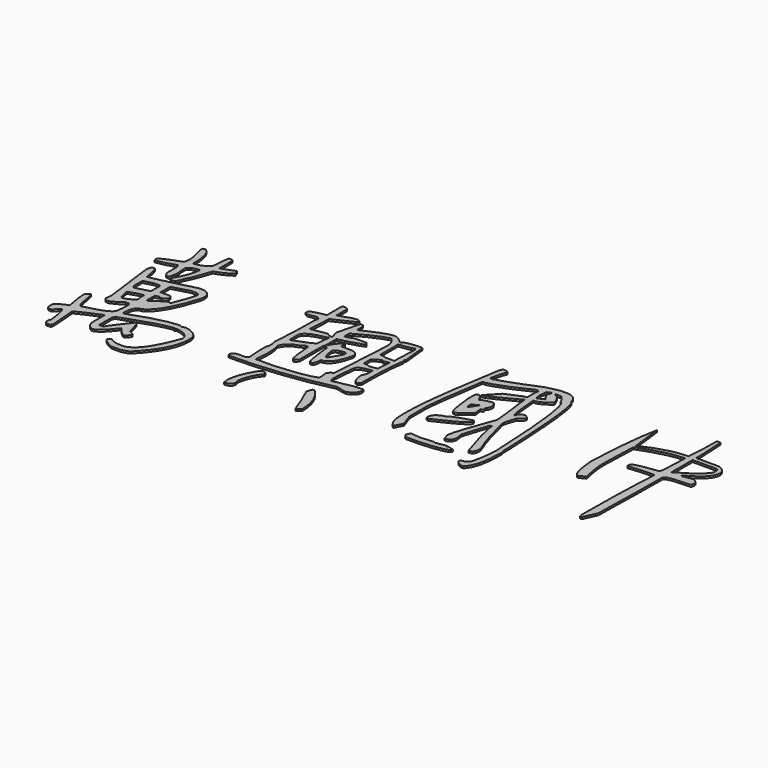
from build123d import *

# Parameters (mm, degrees)
F1_DEPTH = 1


# Not quite as in the source:
# - ends of sketch curves that miss each other by under 0.0002 mm in the source are joined


with BuildPart() as f1:
    # F0 (on Top) → F1 (new body)
    with BuildSketch(Plane.XY):
        with BuildLine():
            Line((-129.622072, 32.734284), (-130.536865, 32.734284))
            add(Edge.make_bspline(
                [(-134.633542, 45.790156), (-131.902424, 44.52872), (-130.536865, 40.176762), (-130.536865, 32.734284)],
                knots=[0, 0, 0, 0, 1, 1, 1, 1], degree=3))
            add(Edge.make_bspline(
                [(-135.786971, 45.269817), (-135.62788, 45.269817), (-135.243404, 45.443263), (-134.633542, 45.790156)],
                knots=[0, 0, 0, 0, 1, 1, 1, 1], degree=3))
            Line((-135.786971, 45.269817), (-135.786971, 44.560262))
            add(Edge.make_bspline(
                [(-133.758523, 34.910264), (-133.758523, 35.604054), (-134.434672, 38.82072), (-135.786971, 44.560262)],
                knots=[0, 0, 0, 0, 1, 1, 1, 1], degree=3))
            Line((-133.758523, 34.910264), (-134.315351, 31.598998))
            add(Edge.make_bspline(
                [(-144.815578, 26.584786), (-144.815578, 27.467788), (-141.315502, 29.139192), (-134.315351, 31.598998)],
                knots=[0, 0, 0, 0, 1, 1, 1, 1], degree=3))
            Line((-144.815578, 26.584786), (-144.815578, 25.307579))
            add(Edge.make_bspline(
                [(-134.474446, 27.767376), (-139.03515, 26.127512), (-142.482194, 25.307579), (-144.815578, 25.307579)],
                knots=[0, 0, 0, 0, 1, 1, 1, 1], degree=3))
            Line((-134.474446, 27.767376), (-133.758523, 26.111743))
            Line((-133.758523, 26.111743), (-133.758523, 19.583812))
            add(Edge.make_bspline(
                [(-132.167581, 17.50244), (-132.538799, 17.50244), (-133.069113, 18.196231), (-133.758523, 19.583812)],
                knots=[0, 0, 0, 0, 1, 1, 1, 1], degree=3))
            Line((-132.167581, 17.50244), (-131.133466, 17.50244))
            add(Edge.make_bspline(
                [(-130.059578, 22.374739), (-130.351253, 19.12654), (-130.709216, 17.50244), (-131.133466, 17.50244)],
                knots=[0, 0, 0, 0, 1, 1, 1, 1], degree=3))
            add(Edge.make_bspline(
                [(-130.536865, 27.199734), (-130.536865, 25.528333), (-130.377769, 23.920001), (-130.059578, 22.374739)],
                knots=[0, 0, 0, 0, 1, 1, 1, 1], degree=3))
            add(Edge.make_bspline(
                [(-124.650376, 30.179878), (-128.574702, 29.580696), (-130.536865, 28.587315), (-130.536865, 27.199734)],
                knots=[0, 0, 0, 0, 1, 1, 1, 1], degree=3))
            add(Edge.make_bspline(
                [(-129.264107, 17.50244), (-126.692084, 21.507502), (-125.154174, 25.733315), (-124.650376, 30.179878)],
                knots=[0, 0, 0, 0, 1, 1, 1, 1], degree=3))
            Line((-129.264107, 17.50244), (-129.264107, 16.367146))
            add(Edge.make_bspline(
                [(-128.03113, 15.752199), (-128.667503, 16.162163), (-129.078495, 16.367146), (-129.264107, 16.367146)],
                knots=[0, 0, 0, 0, 1, 1, 1, 1], degree=3))
            add(Edge.make_bspline(
                [(-124.96856, 19.631116), (-125.604938, 17.045171), (-126.625794, 15.752199), (-128.03113, 15.752199)],
                knots=[0, 0, 0, 0, 1, 1, 1, 1], degree=3))
            add(Edge.make_bspline(
                [(-119.877542, 32.355858), (-121.945771, 26.080207), (-123.642777, 21.838627), (-124.96856, 19.631116)],
                knots=[0, 0, 0, 0, 1, 1, 1, 1], degree=3))
            add(Edge.make_bspline(
                [(-111.485318, 36.471297), (-114.136893, 34.579143), (-116.934301, 33.20733), (-119.877542, 32.355858)],
                knots=[0, 0, 0, 0, 1, 1, 1, 1], degree=3))
            Line((-111.485318, 36.471297), (-112.280789, 38.694573))
            add(Edge.make_bspline(
                [(-119.519584, 36.092863), (-115.117976, 37.827336), (-112.705044, 38.694573), (-112.280789, 38.694573)],
                knots=[0, 0, 0, 0, 1, 1, 1, 1], degree=3))
            Line((-119.519584, 36.092863), (-119.519584, 44.512957))
            add(Edge.make_bspline(
                [(-120.155959, 45.269817), (-119.731709, 45.175209), (-119.519584, 44.922922), (-119.519584, 44.512957)],
                knots=[0, 0, 0, 0, 1, 1, 1, 1], degree=3))
            Line((-120.155959, 45.269817), (-121.62758, 45.269817))
            add(Edge.make_bspline(
                [(-122.701468, 37.37007), (-122.489341, 42.636568), (-122.131378, 45.269817), (-121.62758, 45.269817)],
                knots=[0, 0, 0, 0, 1, 1, 1, 1], degree=3))
            add(Edge.make_bspline(
                [(-129.622072, 32.734284), (-125.008336, 33.7119), (-122.701468, 35.257162), (-122.701468, 37.37007)],
                knots=[0, 0, 0, 0, 1, 1, 1, 1], degree=3))
        make_face()
    extrude(amount=F1_DEPTH)


with BuildPart() as f1b:
    # F0 (on Top) → F1, piece 2 (new body)
    with BuildSketch(Plane.XY):
        with BuildLine():
            Line((-140.20184, 19.583812), (-141.19618, 19.583812))
            add(Edge.make_bspline(
                [(-142.309843, 17.029397), (-141.93862, 18.73234), (-141.567399, 19.583812), (-141.19618, 19.583812)],
                knots=[0, 0, 0, 0, 1, 1, 1, 1], degree=3))
            Line((-142.309843, 17.029397), (-138.809767, -10.40685))
            Line((-138.809767, -10.40685), (-139.287047, -13.386994))
            add(Edge.make_bspline(
                [(-136.701764, -14.711506), (-138.213163, -14.711506), (-139.074924, -14.270002), (-139.287047, -13.386994)],
                knots=[0, 0, 0, 0, 1, 1, 1, 1], degree=3))
            Line((-136.701764, -14.711506), (-132.741804248, -12.6892637488))
            Line((-132.741804248, -12.6892637488), (-130.775501, -11.116414))
            Line((-130.775501, -11.116414), (-129.661846, -11.116414))
            add(Edge.make_bspline(
                [(-128.269766, -12.819351), (-128.269766, -11.68406), (-128.733793, -11.116414), (-129.661846, -11.116414)],
                knots=[0, 0, 0, 0, 1, 1, 1, 1], degree=3))
            Line((-128.269766, -12.819351), (-128.269766, -13.386994))
            add(Edge.make_bspline(
                [(-128.747053, -18.826945), (-128.428862, -16.682501), (-128.269766, -14.869184), (-128.269766, -13.386994)],
                knots=[0, 0, 0, 0, 1, 1, 1, 1], degree=3))
            add(Edge.make_bspline(
                [(-142.826896, -25.260268), (-133.440334, -23.241969), (-128.747053, -21.097527), (-128.747053, -18.826945)],
                knots=[0, 0, 0, 0, 1, 1, 1, 1], degree=3))
            Line((-142.826896, -25.260268), (-144.059873, -23.793852))
            add(Edge.make_bspline(
                [(-146.20765, -14.474984), (-145.756884, -14.474984), (-145.040959, -17.581274), (-144.059873, -23.793852)],
                knots=[0, 0, 0, 0, 1, 1, 1, 1], degree=3))
            Line((-146.20765, -14.474984), (-148.315646, -15.799496))
            add(Edge.make_bspline(
                [(-146.764478, -27.436248), (-147.79859, -22.422039), (-148.315646, -18.543122), (-148.315646, -15.799496)],
                knots=[0, 0, 0, 0, 1, 1, 1, 1], degree=3))
            add(Edge.make_bspline(
                [(-152.849837, -31.362469), (-152.637709, -30.227178), (-150.609256, -28.918437), (-146.764478, -27.436248)],
                knots=[0, 0, 0, 0, 1, 1, 1, 1], degree=3))
            Line((-152.849837, -31.362469), (-152.849837, -33.680362))
            add(Edge.make_bspline(
                [(-150.383875, -35.004874), (-151.815722, -35.004874), (-152.637709, -34.56337), (-152.849837, -33.680362)],
                knots=[0, 0, 0, 0, 1, 1, 1, 1], degree=3))
            Line((-150.383875, -35.004874), (-147.400861, -32.02473))
            add(Edge.make_bspline(
                [(-144.775804, -42.526187), (-145.491725, -35.525215), (-146.366744, -32.02473), (-147.400861, -32.02473)],
                knots=[0, 0, 0, 0, 1, 1, 1, 1], degree=3))
            add(Edge.make_bspline(
                [(-145.332631, -42.6681), (-145.332631, -42.573491), (-145.147022, -42.526187), (-144.775804, -42.526187)],
                knots=[0, 0, 0, 0, 1, 1, 1, 1], degree=3))
            Line((-145.332631, -42.6681), (-145.332631, -44.371037))
            add(Edge.make_bspline(
                [(-144.218969, -45.790157), (-144.53716, -45.790157), (-144.908381, -45.317117), (-145.332631, -44.371037)],
                knots=[0, 0, 0, 0, 1, 1, 1, 1], degree=3))
            Line((-144.218969, -45.790157), (-142.071199, -45.790157))
            add(Edge.make_bspline(
                [(-141.593912, -44.371037), (-141.912104, -45.1279), (-142.071199, -45.60094), (-142.071199, -45.790157)],
                knots=[0, 0, 0, 0, 1, 1, 1, 1], degree=3))
            add(Edge.make_bspline(
                [(-142.628027, -30.842131), (-141.938617, -38.221537), (-141.593912, -42.731172), (-141.593912, -44.371037)],
                knots=[0, 0, 0, 0, 1, 1, 1, 1], degree=3))
            Line((-142.628027, -30.842131), (-142.071199, -30.842131))
            add(Edge.make_bspline(
                [(-130.258447, -25.260268), (-138.133615, -28.571539), (-142.071199, -30.43216), (-142.071199, -30.842131)],
                knots=[0, 0, 0, 0, 1, 1, 1, 1], degree=3))
            Line((-130.258447, -25.260268), (-130.258447, -32.497764))
            add(Edge.make_bspline(
                [(-127.036789, -37.985018), (-129.184561, -36.912794), (-130.258447, -35.083709), (-130.258447, -32.497764)],
                knots=[0, 0, 0, 0, 1, 1, 1, 1], degree=3))
            add(Edge.make_bspline(
                [(-117.61045, -29.990662), (-121.587808, -35.320233), (-124.729921, -37.985018), (-127.036789, -37.985018)],
                knots=[0, 0, 0, 0, 1, 1, 1, 1], degree=3))
            add(Edge.make_bspline(
                [(-112.638754, -34.389918), (-113.858478, -34.389918), (-115.51571, -32.9235), (-117.61045, -29.990662)],
                knots=[0, 0, 0, 0, 1, 1, 1, 1], degree=3))
            Line((-112.638754, -34.389918), (-110.451211, -31.882817))
            add(Edge.make_bspline(
                [(-113.394452, -29.848749), (-111.432291, -30.889432), (-110.451211, -31.567455), (-110.451211, -31.882817)],
                knots=[0, 0, 0, 0, 1, 1, 1, 1], degree=3))
            add(Edge.make_bspline(
                [(-115.621769, -22.80047), (-115.224035, -22.80047), (-114.481596, -25.149897), (-113.394452, -29.848749)],
                knots=[0, 0, 0, 0, 1, 1, 1, 1], degree=3))
            Line((-115.621769, -22.80047), (-116.41724, -22.80047))
            add(Edge.make_bspline(
                [(-124.212863, -33.585754), (-124.212863, -32.828891), (-121.614322, -29.233796), (-116.41724, -22.80047)],
                knots=[0, 0, 0, 0, 1, 1, 1, 1], degree=3))
            Line((-124.212863, -33.585754), (-126.559502, -33.585754))
            Line((-126.559502, -33.585754), (-126.559502, -25.260268))
            Line((-126.559502, -25.260268), (-125.923127, -23.793852))
            add(Edge.make_bspline(
                [(-100.627133, -16.509052), (-104.074177, -16.509052), (-112.506175, -18.937318), (-125.923127, -23.793852)],
                knots=[0, 0, 0, 0, 1, 1, 1, 1], degree=3))
            Line((-100.627133, -16.509052), (-100.627133, -17.076703))
            add(Edge.make_bspline(
                [(-99.593026, -16.509052), (-100.255914, -16.887486), (-100.600617, -17.076703), (-100.627133, -17.076703)],
                knots=[0, 0, 0, 0, 1, 1, 1, 1], degree=3))
            add(Edge.make_bspline(
                [(-92.592874, -21.807089), (-92.592874, -18.968855), (-94.926258, -17.202842), (-99.593026, -16.509052)],
                knots=[0, 0, 0, 0, 1, 1, 1, 1], degree=3))
            add(Edge.make_bspline(
                [(-108.06479, -41.958544), (-102.523006, -41.958544), (-97.365701, -35.241393), (-92.592874, -21.807089)],
                knots=[0, 0, 0, 0, 1, 1, 1, 1], degree=3))
            add(Edge.make_bspline(
                [(-114.66721, -40.113686), (-113.049747, -41.343591), (-110.84894, -41.958544), (-108.06479, -41.958544)],
                knots=[0, 0, 0, 0, 1, 1, 1, 1], degree=3))
            add(Edge.make_bspline(
                [(-116.178604, -41.438197), (-116.178604, -40.744407), (-115.674806, -40.302903), (-114.66721, -40.113686)],
                knots=[0, 0, 0, 0, 1, 1, 1, 1], degree=3))
            add(Edge.make_bspline(
                [(-111.008038, -45.175202), (-114.216439, -43.693018), (-115.93996, -42.44735), (-116.178604, -41.438197)],
                knots=[0, 0, 0, 0, 1, 1, 1, 1], degree=3))
            Line((-111.008038, -45.175202), (-106.553396, -45.175202))
            add(Edge.make_bspline(
                [(-102.218075, -44.039907), (-104.286304, -44.79677), (-105.731411, -45.175202), (-106.553396, -45.175202)],
                knots=[0, 0, 0, 0, 1, 1, 1, 1], degree=3))
            add(Edge.make_bspline(
                [(-89.888269, -20.577186), (-89.888269, -27.956592), (-93.998205, -35.777499), (-102.218075, -44.039907)],
                knots=[0, 0, 0, 0, 1, 1, 1, 1], degree=3))
            Line((-89.888269, -20.577186), (-89.888269, -19.962239))
            add(Edge.make_bspline(
                [(-97.56457, -13.292386), (-92.447036, -14.270002), (-89.888269, -16.493286), (-89.888269, -19.962239)],
                knots=[0, 0, 0, 0, 1, 1, 1, 1], degree=3))
            add(Edge.make_bspline(
                [(-98.996417, -13.907341), (-98.307012, -13.497371), (-97.82973, -13.292386), (-97.56457, -13.292386)],
                knots=[0, 0, 0, 0, 1, 1, 1, 1], degree=3))
            add(Edge.make_bspline(
                [(-100.547585, -13.292386), (-100.229399, -13.292386), (-99.712342, -13.497371), (-98.996417, -13.907341)],
                knots=[0, 0, 0, 0, 1, 1, 1, 1], degree=3))
            add(Edge.make_bspline(
                [(-124.531054, -19.252674), (-113.686124, -15.279149), (-105.691635, -13.292386), (-100.547585, -13.292386)],
                knots=[0, 0, 0, 0, 1, 1, 1, 1], degree=3))
            Line((-124.531054, -19.252674), (-125.525395, -19.252674))
            add(Edge.make_bspline(
                [(-121.707128, -11.731361), (-124.252639, -11.731361), (-125.525395, -14.238466), (-125.525395, -19.252674)],
                knots=[0, 0, 0, 0, 1, 1, 1, 1], degree=3))
            add(Edge.make_bspline(
                [(-108.462529, 11.211021), (-112.174728, -1.403347), (-116.589594, -9.050808), (-121.707128, -11.731361)],
                knots=[0, 0, 0, 0, 1, 1, 1, 1], degree=3))
            Line((-108.462529, 11.211021), (-108.462529, 12.299011))
            add(Edge.make_bspline(
                [(-112.59898, 17.17131), (-109.841346, 16.698273), (-108.462529, 15.074173), (-108.462529, 12.299011)],
                knots=[0, 0, 0, 0, 1, 1, 1, 1], degree=3))
            Line((-112.59898, 17.17131), (-115.064942, 17.17131))
            add(Edge.make_bspline(
                [(-138.014296, 11.825968), (-136.396838, 11.825968), (-128.747053, 13.607749), (-115.064942, 17.17131)],
                knots=[0, 0, 0, 0, 1, 1, 1, 1], degree=3))
            add(Edge.make_bspline(
                [(-140.20184, 19.583812), (-139.432882, 19.583812), (-138.703701, 16.997864), (-138.014296, 11.825968)],
                knots=[0, 0, 0, 0, 1, 1, 1, 1], degree=3))
        make_face()
        with BuildLine():
            add(Edge.make_bspline(
                [(-136.105162, -3.547788), (-135.574848, -7.237494), (-134.911955, -9.082347), (-134.116481, -9.082347)],
                knots=[0, 0, 0, 0, 1, 1, 1, 1], degree=3))
            add(Edge.make_bspline(
                [(-128.747053, -1.561025), (-129.860713, -1.561025), (-132.313416, -2.223279), (-136.105162, -3.547788)],
                knots=[0, 0, 0, 0, 1, 1, 1, 1], degree=3))
            add(Edge.make_bspline(
                [(-128.150444, -5.676464), (-128.548183, -4.951137), (-128.747053, -3.579324), (-128.747053, -1.561025)],
                knots=[0, 0, 0, 0, 1, 1, 1, 1], degree=3))
            add(Edge.make_bspline(
                [(-134.116481, -9.082347), (-131.305815, -8.293948), (-129.317136, -7.158653), (-128.150444, -5.676464)],
                knots=[0, 0, 0, 0, 1, 1, 1, 1], degree=3))
        make_face(mode=Mode.SUBTRACT)
        with BuildLine():
            Line((-137.099503, 2.696327), (-137.099503, 7.899747))
            Line((-137.099503, 7.899747), (-132.207355, 9.176954))
            Line((-132.207355, 9.176954), (-128.747053, 9.176954))
            Line((-128.747053, 9.176954), (-128.747053, 2.980144))
            Line((-128.747053, 2.980144), (-135.627883, 1.040685))
            add(Edge.make_bspline(
                [(-137.099503, 2.696327), (-136.913892, 1.592566), (-136.423351, 1.040685), (-135.627883, 1.040685)],
                knots=[0, 0, 0, 0, 1, 1, 1, 1], degree=3))
        make_face(mode=Mode.SUBTRACT)
        with BuildLine():
            Line((-125.008334, 4.635785), (-125.008334, 10.879891))
            Line((-125.008334, 10.879891), (-116.099056, 13.339697))
            Line((-116.099056, 13.339697), (-112.99672, 13.339697))
            Line((-112.99672, 13.339697), (-111.684188, 12.582837))
            add(Edge.make_bspline(
                [(-115.820639, -0.141914), (-113.063005, 6.669847), (-111.684188, 10.91143), (-111.684188, 12.582837)],
                knots=[0, 0, 0, 0, 1, 1, 1, 1], degree=3))
            Line((-115.820639, -0.141914), (-117.61045, -0.141914))
            add(Edge.make_bspline(
                [(-124.013993, -4.351952), (-120.222247, -1.54526), (-118.087733, -0.141914), (-117.61045, -0.141914)],
                knots=[0, 0, 0, 0, 1, 1, 1, 1], degree=3))
            Line((-124.013993, -4.351952), (-125.008334, -4.351952))
            Line((-125.008334, -4.351952), (-125.008334, 0.804172))
            add(Edge.make_bspline(
                [(-123.099208, 1.466424), (-123.815128, 1.024923), (-124.451504, 0.804172), (-125.008334, 0.804172)],
                knots=[0, 0, 0, 0, 1, 1, 1, 1], degree=3))
            Line((-123.099208, 1.466424), (-122.025319, 0.804172))
            add(Edge.make_bspline(
                [(-119.002523, 2.838231), (-119.453294, 1.482192), (-120.460893, 0.804172), (-122.025319, 0.804172)],
                knots=[0, 0, 0, 0, 1, 1, 1, 1], degree=3))
            Line((-119.002523, 2.838231), (-119.002523, 3.263969))
            add(Edge.make_bspline(
                [(-120.116186, 4.635785), (-119.771483, 4.635785), (-119.400262, 4.178513), (-119.002523, 3.263969)],
                knots=[0, 0, 0, 0, 1, 1, 1, 1], degree=3))
            Line((-120.116186, 4.635785), (-125.008334, 4.635785))
        make_face(mode=Mode.SUBTRACT)
    extrude(amount=F1_DEPTH)


with BuildPart() as f1c:
    # F0 (on Top) → F1, piece 3 (new body)
    with BuildSketch(Plane.XY):
        with BuildLine():
            Line((-56.319381, 33.443848), (-56.319381, 40.066388))
            add(Edge.make_bspline(
                [(-58.984204, 41.3909), (-57.207655, 41.170147), (-56.319381, 40.728643), (-56.319381, 40.066388)],
                knots=[0, 0, 0, 0, 1, 1, 1, 1], degree=3))
            add(Edge.make_bspline(
                [(-59.541039, 40.63404), (-59.461491, 41.138613), (-59.27588, 41.3909), (-58.984204, 41.3909)],
                knots=[0, 0, 0, 0, 1, 1, 1, 1], degree=3))
            Line((-59.541039, 40.63404), (-59.541039, 31.267868))
            add(Edge.make_bspline(
                [(-67.575298, 28.713462), (-67.575298, 29.501856), (-64.897212, 30.353324), (-59.541039, 31.267868)],
                knots=[0, 0, 0, 0, 1, 1, 1, 1], degree=3))
            Line((-67.575298, 28.713462), (-67.575298, 27.388951))
            add(Edge.make_bspline(
                [(-66.382095, 26.773995), (-67.044984, 27.183965), (-67.442718, 27.388951), (-67.575298, 27.388951)],
                knots=[0, 0, 0, 0, 1, 1, 1, 1], degree=3))
            add(Edge.make_bspline(
                [(-61.370617, 27.388951), (-61.87442, 27.388951), (-63.544913, 27.183965), (-66.382095, 26.773995)],
                knots=[0, 0, 0, 0, 1, 1, 1, 1], degree=3))
            Line((-61.370617, 27.388951), (-59.938771, 26.490178))
            Line((-59.938771, 26.490178), (-60.535372, 25.023753))
            Line((-60.535372, 25.023753), (-60.535372, 23.935763))
            add(Edge.make_bspline(
                [(-61.529713, -0.425731), (-60.866819, 7.016748), (-60.535372, 15.137246), (-60.535372, 23.935763)],
                knots=[0, 0, 0, 0, 1, 1, 1, 1], degree=3))
            add(Edge.make_bspline(
                [(-61.052433, -2.459798), (-61.052433, -1.892152), (-61.211527, -1.21413), (-61.529713, -0.425731)],
                knots=[0, 0, 0, 0, 1, 1, 1, 1], degree=3))
            Line((-61.052433, -2.459798), (-61.012659, -4.730387))
            add(Edge.make_bspline(
                [(-61.529713, -7.142888), (-61.529713, -6.322953), (-61.357362, -5.518786), (-61.012659, -4.730387)],
                knots=[0, 0, 0, 0, 1, 1, 1, 1], degree=3))
            Line((-61.529713, -7.142888), (-61.529713, -10.123033))
            Line((-61.529713, -10.123033), (-61.052433, -17.549737))
            Line((-61.052433, -17.549737), (-62.364958, -18.353902))
            Line((-62.364958, -18.353902), (-65.984356, -18.353902))
            add(Edge.make_bspline(
                [(-69.086692, -20.387969), (-68.60941, -19.031924), (-67.575298, -18.353902), (-65.984356, -18.353902)],
                knots=[0, 0, 0, 0, 1, 1, 1, 1], degree=3))
            Line((-69.086692, -20.387969), (-68.728734, -21.570568))
            add(Edge.make_bspline(
                [(-16.744674, -15.610279), (-33.979888, -19.583805), (-51.307908, -21.570568), (-68.728734, -21.570568)],
                knots=[0, 0, 0, 0, 1, 1, 1, 1], degree=3))
            add(Edge.make_bspline(
                [(-11.255917, -16.792877), (-12.024874, -16.792877), (-13.85446, -16.398678), (-16.744674, -15.610279)],
                knots=[0, 0, 0, 0, 1, 1, 1, 1], degree=3))
            add(Edge.make_bspline(
                [(-6.602412, -11.920579), (-6.602412, -14.159625), (-8.15358, -15.783725), (-11.255917, -16.792877)],
                knots=[0, 0, 0, 0, 1, 1, 1, 1], degree=3))
            Line((-6.602412, -11.920579), (-6.96037, -10.596067))
            add(Edge.make_bspline(
                [(-21.99478, -13.055873), (-14.941602, -11.416002), (-9.930132, -10.596067), (-6.96037, -10.596067)],
                knots=[0, 0, 0, 0, 1, 1, 1, 1], degree=3))
            Line((-21.99478, -13.055873), (-22.670937, -11.400231))
            add(Edge.make_bspline(
                [(-21.676596, 1.277206), (-22.33949, -3.705466), (-22.670937, -7.931279), (-22.670937, -11.400231)],
                knots=[0, 0, 0, 0, 1, 1, 1, 1], degree=3))
            add(Edge.make_bspline(
                [(-14.318487, 4.730394), (-19.223893, 4.099676), (-21.676596, 2.948613), (-21.676596, 1.277206)],
                knots=[0, 0, 0, 0, 1, 1, 1, 1], degree=3))
            Line((-14.318487, 4.730394), (-14.318487, 2.459805))
            add(Edge.make_bspline(
                [(-15.352594, -1.277199), (-14.663189, 0.015773), (-14.318487, 1.261441), (-14.318487, 2.459805)],
                knots=[0, 0, 0, 0, 1, 1, 1, 1], degree=3))
            add(Edge.make_bspline(
                [(-12.727545, -7.80514), (-14.477578, -7.205958), (-15.352594, -5.029978), (-15.352594, -1.277199)],
                knots=[0, 0, 0, 0, 1, 1, 1, 1], degree=3))
            add(Edge.make_bspline(
                [(-11.136595, -6.527932), (-11.136595, -6.906367), (-11.666912, -7.332103), (-12.727545, -7.80514)],
                knots=[0, 0, 0, 0, 1, 1, 1, 1], degree=3))
            Line((-11.136595, -6.527932), (-11.136595, -4.162735))
            add(Edge.make_bspline(
                [(-9.704749, 18.685039), (-10.659313, 13.481607), (-11.136595, 5.865682), (-11.136595, -4.162735)],
                knots=[0, 0, 0, 0, 1, 1, 1, 1], degree=3))
            add(Edge.make_bspline(
                [(-10.102488, 20.246063), (-10.102488, 19.20538), (-9.969908, 18.685039), (-9.704749, 18.685039)],
                knots=[0, 0, 0, 0, 1, 1, 1, 1], degree=3))
            add(Edge.make_bspline(
                [(-9.625201, 20.387976), (-9.625201, 20.293367), (-9.784296, 20.246063), (-10.102488, 20.246063)],
                knots=[0, 0, 0, 0, 1, 1, 1, 1], degree=3))
            Line((-9.625201, 20.387976), (-10.937733, 33.01811))
            add(Edge.make_bspline(
                [(-21.318631, 31.125955), (-19.674657, 32.387391), (-16.214357, 33.01811), (-10.937733, 33.01811)],
                knots=[0, 0, 0, 0, 1, 1, 1, 1], degree=3))
            add(Edge.make_bspline(
                [(-26.290327, 34.200708), (-25.123635, 34.200708), (-23.466403, 33.17579), (-21.318631, 31.125955)],
                knots=[0, 0, 0, 0, 1, 1, 1, 1], degree=3))
            add(Edge.make_bspline(
                [(-41.76225, 28.618854), (-34.205269, 32.34009), (-29.047961, 34.200708), (-26.290327, 34.200708)],
                knots=[0, 0, 0, 0, 1, 1, 1, 1], degree=3))
            Line((-41.76225, 28.618854), (-41.76225, 32.166641))
            add(Edge.make_bspline(
                [(-42.875913, 33.585761), (-42.557721, 33.585761), (-42.186501, 33.112721), (-41.76225, 32.166641)],
                knots=[0, 0, 0, 0, 1, 1, 1, 1], degree=3))
            Line((-42.875913, 33.585761), (-43.870246, 33.585761))
            add(Edge.make_bspline(
                [(-46.97259, 21.475966), (-45.116488, 29.549163), (-44.082374, 33.585761), (-43.870246, 33.585761)],
                knots=[0, 0, 0, 0, 1, 1, 1, 1], degree=3))
            Line((-46.97259, 21.475966), (-46.5306612376, 19.7099567259))
            Line((-46.5306612376, 19.7099567259), (-45.978249, 18.685039))
            Line((-45.978249, 18.685039), (-45.978249, 17.50244))
            add(Edge.make_bspline(
                [(-49.001038, 18.685039), (-47.913894, 17.89664), (-46.906298, 17.50244), (-45.978249, 17.50244)],
                knots=[0, 0, 0, 0, 1, 1, 1, 1], degree=3))
            add(Edge.make_bspline(
                [(-56.398921, 17.50244), (-51.78519, 18.290839), (-49.319229, 18.685039), (-49.001038, 18.685039)],
                knots=[0, 0, 0, 0, 1, 1, 1, 1], degree=3))
            Line((-56.398921, 17.50244), (-57.393262, 17.50244))
            Line((-57.393262, 17.50244), (-56.836434, 25.118362))
            Line((-56.836434, 25.118362), (-56.836434, 29.044584))
            add(Edge.make_bspline(
                [(-45.262326, 34.673751), (-45.262326, 34.421462), (-49.120362, 32.545072), (-56.836434, 29.044584)],
                knots=[0, 0, 0, 0, 1, 1, 1, 1], degree=3))
            add(Edge.make_bspline(
                [(-46.932816, 35.998254), (-45.819156, 35.493681), (-45.262326, 35.05218), (-45.262326, 34.673751)],
                knots=[0, 0, 0, 0, 1, 1, 1, 1], degree=3))
            add(Edge.make_bspline(
                [(-56.319381, 33.443848), (-51.546549, 35.146785), (-48.417694, 35.998254), (-46.932816, 35.998254)],
                knots=[0, 0, 0, 0, 1, 1, 1, 1], degree=3))
        make_face()
        with BuildLine():
            Line((-41.284963, 21.050227), (-42.279304, 21.050227))
            Line((-42.279304, 21.050227), (-42.279304, 24.219589))
            add(Edge.make_bspline(
                [(-26.171013, 31.598998), (-30.333977, 30.526773), (-35.703408, 28.06697), (-42.279304, 24.219589)],
                knots=[0, 0, 0, 0, 1, 1, 1, 1], degree=3))
            add(Edge.make_bspline(
                [(-23.38686, 26.300961), (-23.38686, 28.003898), (-24.314911, 29.76991), (-26.171013, 31.598998)],
                knots=[0, 0, 0, 0, 1, 1, 1, 1], degree=3))
            add(Edge.make_bspline(
                [(-25.415308, -7.000975), (-24.063009, 10.186101), (-23.38686, 21.286746), (-23.38686, 26.300961)],
                knots=[0, 0, 0, 0, 1, 1, 1, 1], degree=3))
            add(Edge.make_bspline(
                [(-27.881269, -9.035043), (-27.032769, -7.678998), (-26.210782, -7.000975), (-25.415308, -7.000975)],
                knots=[0, 0, 0, 0, 1, 1, 1, 1], degree=3))
            Line((-27.881269, -9.035043), (-27.403989, -13.055873))
            add(Edge.make_bspline(
                [(-48.404436, -17.171303), (-34.404138, -16.067548), (-27.403989, -14.695738), (-27.403989, -13.055873)],
                knots=[0, 0, 0, 0, 1, 1, 1, 1], degree=3))
            Line((-48.404436, -17.171303), (-57.830775, -17.171303))
            add(Edge.make_bspline(
                [(-57.353488, -10.643371), (-57.671679, -14.14386), (-57.830775, -16.319837), (-57.830775, -17.171303)],
                knots=[0, 0, 0, 0, 1, 1, 1, 1], degree=3))
            add(Edge.make_bspline(
                [(-58.347829, -2.365189), (-57.684935, -4.541169), (-57.353488, -7.300563), (-57.353488, -10.643371)],
                knots=[0, 0, 0, 0, 1, 1, 1, 1], degree=3))
            add(Edge.make_bspline(
                [(-54.569343, 2.270588), (-56.504988, 0.819935), (-57.764483, -0.725325), (-58.347829, -2.365189)],
                knots=[0, 0, 0, 0, 1, 1, 1, 1], degree=3))
            add(Edge.make_bspline(
                [(-49.518099, 4.68309), (-50.446147, 3.863154), (-52.129895, 3.058987), (-54.569343, 2.270588)],
                knots=[0, 0, 0, 0, 1, 1, 1, 1], degree=3))
            Line((-49.518099, 4.68309), (-48.046471, 4.68309))
            add(Edge.make_bspline(
                [(-45.898701, -7.852444), (-46.588111, -7.852444), (-47.304034, -3.673933), (-48.046471, 4.68309)],
                knots=[0, 0, 0, 0, 1, 1, 1, 1], degree=3))
            Line((-45.898701, -7.852444), (-45.500962, -7.852444))
            add(Edge.make_bspline(
                [(-43.750932, -5.912985), (-43.750932, -6.354486), (-44.334275, -7.000972), (-45.500962, -7.852444)],
                knots=[0, 0, 0, 0, 1, 1, 1, 1], degree=3))
            Line((-43.750932, -5.912985), (-43.750932, 9.79191))
            add(Edge.make_bspline(
                [(-41.523607, 8.845824), (-42.027405, 8.845824), (-42.769847, 9.161186), (-43.750932, 9.79191)],
                knots=[0, 0, 0, 0, 1, 1, 1, 1], degree=3))
            add(Edge.make_bspline(
                [(-38.858776, -5.439942), (-39.707282, -5.439942), (-40.595558, -0.67802), (-41.523607, 8.845824)],
                knots=[0, 0, 0, 0, 1, 1, 1, 1], degree=3))
            Line((-38.858776, -5.439942), (-38.341722, -5.439942))
            add(Edge.make_bspline(
                [(-36.711006, -1.277199), (-36.711006, -4.052361), (-37.254578, -5.439942), (-38.341722, -5.439942)],
                knots=[0, 0, 0, 0, 1, 1, 1, 1], degree=3))
            add(Edge.make_bspline(
                [(-28.716514, 9.649997), (-30.493068, 2.365199), (-33.157899, -1.277199), (-36.711006, -1.277199)],
                knots=[0, 0, 0, 0, 1, 1, 1, 1], degree=3))
            add(Edge.make_bspline(
                [(-32.296138, 13.292393), (-29.909722, 13.040103), (-28.716514, 11.825971), (-28.716514, 9.649997)],
                knots=[0, 0, 0, 0, 1, 1, 1, 1], degree=3))
            Line((-32.296138, 13.292393), (-37.745121, 13.292393))
            Line((-37.745121, 13.292393), (-37.745121, 14.474991))
            Line((-37.745121, 14.474991), (-37.387156, 15.373764))
            Line((-37.387156, 15.373764), (-37.943983, 15.704894))
            add(Edge.make_bspline(
                [(-43.273645, 9.79191), (-41.152388, 13.7339), (-39.375835, 15.704894), (-37.943983, 15.704894)],
                knots=[0, 0, 0, 0, 1, 1, 1, 1], degree=3))
            Line((-43.273645, 9.79191), (-43.273645, 17.218614))
            add(Edge.make_bspline(
                [(-33.767758, 19.67842), (-39.229999, 18.03855), (-42.398628, 17.218614), (-43.273645, 17.218614)],
                knots=[0, 0, 0, 0, 1, 1, 1, 1], degree=3))
            Line((-33.767758, 19.67842), (-30.705196, 20.86101))
            add(Edge.make_bspline(
                [(-31.818858, 22.28013), (-31.500667, 22.28013), (-31.129446, 21.80709), (-30.705196, 20.86101)],
                knots=[0, 0, 0, 0, 1, 1, 1, 1], degree=3))
            Line((-31.818858, 22.28013), (-36.830328, 22.28013))
            add(Edge.make_bspline(
                [(-41.284963, 21.050227), (-39.110675, 21.870163), (-37.625797, 22.28013), (-36.830328, 22.28013)],
                knots=[0, 0, 0, 0, 1, 1, 1, 1], degree=3))
        make_face(mode=Mode.SUBTRACT)
        with BuildLine():
            Line((-56.915982, 4.919602), (-57.830775, 4.919602))
            Line((-57.830775, 4.919602), (-57.830775, 10.21764))
            add(Edge.make_bspline(
                [(-46.415755, 16.130624), (-54.025768, 14.743043), (-57.830775, 12.772048), (-57.830775, 10.21764)],
                knots=[0, 0, 0, 0, 1, 1, 1, 1], degree=3))
            Line((-46.415755, 16.130624), (-46.97259, 9.555388))
            add(Edge.make_bspline(
                [(-56.915982, 4.919602), (-50.287054, 7.2848), (-46.97259, 8.830062), (-46.97259, 9.555388)],
                knots=[0, 0, 0, 0, 1, 1, 1, 1], degree=3))
        make_face(mode=Mode.SUBTRACT)
        with BuildLine():
            Line((-32.41546, 8.230877), (-36.114405, 1.986762))
            add(Edge.make_bspline(
                [(-38.262175, 7.947051), (-37.890956, 3.973525), (-37.175033, 1.986762), (-36.114405, 1.986762)],
                knots=[0, 0, 0, 0, 1, 1, 1, 1], degree=3))
            add(Edge.make_bspline(
                [(-33.807532, 10.075727), (-35.796213, 10.075727), (-37.281094, 9.366168), (-38.262175, 7.947051)],
                knots=[0, 0, 0, 0, 1, 1, 1, 1], degree=3))
            Line((-33.807532, 10.075727), (-32.41546, 10.075727))
            Line((-32.41546, 10.075727), (-32.41546, 8.230877))
        make_face(mode=Mode.SUBTRACT)
        with BuildLine():
            Line((-21.159535, 7.332104), (-21.159535, 11.400238))
            add(Edge.make_bspline(
                [(-16.863996, 14.427687), (-19.727689, 13.26086), (-21.159535, 12.25171), (-21.159535, 11.400238)],
                knots=[0, 0, 0, 0, 1, 1, 1, 1], degree=3))
            add(Edge.make_bspline(
                [(-16.744674, 13.623523), (-16.824222, 13.623523), (-16.863996, 13.891578), (-16.863996, 14.427687)],
                knots=[0, 0, 0, 0, 1, 1, 1, 1], degree=3))
            Line((-16.744674, 13.623523), (-13.324146, 14.380383))
            add(Edge.make_bspline(
                [(-13.8412, 7.332104), (-13.8412, 8.120503), (-13.668849, 10.469929), (-13.324146, 14.380383)],
                knots=[0, 0, 0, 0, 1, 1, 1, 1], degree=3))
            Line((-13.8412, 7.332104), (-17.818555, 6.717157))
            add(Edge.make_bspline(
                [(-21.159535, 7.332104), (-19.462534, 7.332104), (-18.348874, 7.127122), (-17.818555, 6.717157)],
                knots=[0, 0, 0, 0, 1, 1, 1, 1], degree=3))
        make_face(mode=Mode.SUBTRACT)
        with BuildLine():
            Line((-20.682255, 17.549745), (-20.682255, 29.139192))
            add(Edge.make_bspline(
                [(-12.846859, 30.700225), (-13.615817, 30.195646), (-16.227615, 29.675302), (-20.682255, 29.139192)],
                knots=[0, 0, 0, 0, 1, 1, 1, 1], degree=3))
            add(Edge.make_bspline(
                [(-12.329805, 29.801444), (-12.674508, 29.801444), (-12.846859, 30.101037), (-12.846859, 30.700225)],
                knots=[0, 0, 0, 0, 1, 1, 1, 1], degree=3))
            add(Edge.make_bspline(
                [(-12.886633, 16.887484), (-12.515415, 22.563953), (-12.329805, 26.868606), (-12.329805, 29.801444)],
                knots=[0, 0, 0, 0, 1, 1, 1, 1], degree=3))
            Line((-12.886633, 16.887484), (-16.784448, 16.887484))
            Line((-16.784448, 16.887484), (-20.682255, 17.549745))
        make_face(mode=Mode.SUBTRACT)
    extrude(amount=F1_DEPTH)


with BuildPart() as f1d:
    # F0 (on Top) → F1, piece 4 (new body)
    with BuildSketch(Plane.XY):
        with BuildLine():
            Line((-47.887383, -23.746548), (-49.319229, -23.746548))
            Line((-49.319229, -23.746548), (-50.1147, -24.219582))
            add(Edge.make_bspline(
                [(-55.523902, -38.789183), (-55.523902, -34.815657), (-53.720835, -29.959123), (-50.1147, -24.219582)],
                knots=[0, 0, 0, 0, 1, 1, 1, 1], degree=3))
            Line((-55.523902, -38.789183), (-55.165944, -41.296284))
            add(Edge.make_bspline(
                [(-51.307911, -38.268835), (-51.307911, -40.287135), (-52.593922, -41.296284), (-55.165944, -41.296284)],
                knots=[0, 0, 0, 0, 1, 1, 1, 1], degree=3))
            add(Edge.make_bspline(
                [(-51.78519, -36.329377), (-51.78519, -36.865486), (-51.626097, -37.511973), (-51.307911, -38.268835)],
                knots=[0, 0, 0, 0, 1, 1, 1, 1], degree=3))
            add(Edge.make_bspline(
                [(-46.77372, -25.402181), (-49.266195, -28.019662), (-50.936685, -31.66206), (-51.78519, -36.329377)],
                knots=[0, 0, 0, 0, 1, 1, 1, 1], degree=3))
            Line((-46.77372, -25.402181), (-46.77372, -25.165659))
            add(Edge.make_bspline(
                [(-47.887383, -23.746548), (-47.569191, -23.746548), (-47.197971, -24.219585), (-46.77372, -25.165659)],
                knots=[0, 0, 0, 0, 1, 1, 1, 1], degree=3))
        make_face()
    extrude(amount=F1_DEPTH)


with BuildPart() as f1e:
    # F0 (on Top) → F1, piece 5 (new body)
    with BuildSketch(Plane.XY):
        with BuildLine():
            Line((-21.91524, -23.746548), (-22.750485, -23.746548))
            add(Edge.make_bspline(
                [(-23.903914, -26.726692), (-23.612243, -24.739929), (-23.227767, -23.746548), (-22.750485, -23.746548)],
                knots=[0, 0, 0, 0, 1, 1, 1, 1], degree=3))
            add(Edge.make_bspline(
                [(-17.977651, -41.296284), (-19.780721, -36.282075), (-21.756142, -31.425545), (-23.903914, -26.726692)],
                knots=[0, 0, 0, 0, 1, 1, 1, 1], degree=3))
            add(Edge.make_bspline(
                [(-15.631012, -39.73526), (-16.744672, -40.775943), (-17.526885, -41.296284), (-17.977651, -41.296284)],
                knots=[0, 0, 0, 0, 1, 1, 1, 1], degree=3))
            add(Edge.make_bspline(
                [(-21.91524, -23.746548), (-17.725754, -27.720074), (-15.631012, -33.049644), (-15.631012, -39.73526)],
                knots=[0, 0, 0, 0, 1, 1, 1, 1], degree=3))
        make_face()
    extrude(amount=F1_DEPTH)


with BuildPart() as f1f:
    # F0 (on Top) → F1, piece 6 (new body)
    with BuildSketch(Plane.XY):
        with BuildLine():
            Line((28.5972, 29.328409), (27.20512, 29.328409))
            add(Edge.make_bspline(
                [(29.511993, 37.606591), (28.58394, 35.777503), (27.814982, 33.01811), (27.20512, 29.328409)],
                knots=[0, 0, 0, 0, 1, 1, 1, 1], degree=3))
            add(Edge.make_bspline(
                [(26.250561, 38.694573), (28.424849, 38.59997), (29.511993, 38.237309), (29.511993, 37.606591)],
                knots=[0, 0, 0, 0, 1, 1, 1, 1], degree=3))
            add(Edge.make_bspline(
                [(25.813048, 37.653896), (26.104723, 37.622371), (26.250561, 37.969263), (26.250561, 38.694573)],
                knots=[0, 0, 0, 0, 1, 1, 1, 1], degree=3))
            add(Edge.make_bspline(
                [(19.290183, -13.812733), (19.290183, -5.550319), (21.464471, 11.605224), (25.813048, 37.653896)],
                knots=[0, 0, 0, 0, 1, 1, 1, 1], degree=3))
            Line((19.290183, -13.812733), (19.290183, -18.306597))
            add(Edge.make_bspline(
                [(22.591389, -28.240412), (20.390585, -26.505939), (19.290183, -23.194667), (19.290183, -18.306597)],
                knots=[0, 0, 0, 0, 1, 1, 1, 1], degree=3))
            Line((22.591389, -28.240412), (24.858481, -23.793852))
            add(Edge.make_bspline(
                [(22.591389, -17.123999), (22.591389, -17.817789), (23.347086, -20.041074), (24.858481, -23.793852)],
                knots=[0, 0, 0, 0, 1, 1, 1, 1], degree=3))
            Line((22.591389, -17.123999), (22.591389, -5.534551))
            add(Edge.make_bspline(
                [(26.767614, 24.881841), (23.983464, 6.811763), (22.591389, -3.327035), (22.591389, -5.534551)],
                knots=[0, 0, 0, 0, 1, 1, 1, 1], degree=3))
            add(Edge.make_bspline(
                [(48.603306, 33.160022), (37.175031, 27.641234), (29.896467, 24.881841), (26.767614, 24.881841)],
                knots=[0, 0, 0, 0, 1, 1, 1, 1], degree=3))
            add(Edge.make_bspline(
                [(49.995379, 32.59238), (49.385517, 32.970808), (48.921493, 33.160022), (48.603306, 33.160022)],
                knots=[0, 0, 0, 0, 1, 1, 1, 1], degree=3))
            Line((49.995379, 32.59238), (49.518099, 31.50439))
            Line((49.518099, 31.50439), (49.518099, 25.402188))
            Line((49.518099, 25.402188), (48.126027, 25.402188))
            Line((48.126027, 25.402188), (39.7618406848, 21.8199565158))
            Line((39.7618406848, 21.8199565158), (33.727992, 15.468373))
            add(Edge.make_bspline(
                [(49.995379, 23.226208), (40.555785, 18.054318), (35.133322, 15.468373), (33.727992, 15.468373)],
                knots=[0, 0, 0, 0, 1, 1, 1, 1], degree=3))
            add(Edge.make_bspline(
                [(52.342018, 3.311274), (52.342018, 4.793463), (51.559805, 11.431775), (49.995379, 23.226208)],
                knots=[0, 0, 0, 0, 1, 1, 1, 1], degree=3))
            Line((52.342018, 3.311274), (52.342018, 2.223284))
            add(Edge.make_bspline(
                [(44.904361, -21.050229), (44.904361, -18.685032), (47.38358, -10.927194), (52.342018, 2.223284)],
                knots=[0, 0, 0, 0, 1, 1, 1, 1], degree=3))
            add(Edge.make_bspline(
                [(45.819154, -23.793852), (45.819154, -23.131598), (45.514223, -22.217057), (44.904361, -21.050229)],
                knots=[0, 0, 0, 0, 1, 1, 1, 1], degree=3))
            add(Edge.make_bspline(
                [(49.518099, -19.914935), (49.518099, -22.50088), (48.285117, -23.793852), (45.819154, -23.793852)],
                knots=[0, 0, 0, 0, 1, 1, 1, 1], degree=3))
            Line((49.518099, -19.914935), (49.040812, -16.60366))
            Line((49.040812, -16.60366), (53.256811, -3.358571))
            Line((53.256811, -3.358571), (54.211378, -3.358571))
            add(Edge.make_bspline(
                [(60.217189, -26.017136), (56.213315, -13.812733), (54.211378, -6.259878), (54.211378, -3.358571)],
                knots=[0, 0, 0, 0, 1, 1, 1, 1], degree=3))
            add(Edge.make_bspline(
                [(63.001341, -22.705862), (63.001341, -24.913378), (62.07329, -26.017136), (60.217189, -26.017136)],
                knots=[0, 0, 0, 0, 1, 1, 1, 1], degree=3))
            Line((63.001341, -22.705862), (63.001341, -21.570568))
            add(Edge.make_bspline(
                [(56.040964, 1.135294), (58.2948, -8.451623), (60.614925, -16.020243), (63.001341, -21.570568)],
                knots=[0, 0, 0, 0, 1, 1, 1, 1], degree=3))
            add(Edge.make_bspline(
                [(57.910323, 8.230877), (56.664083, 5.04575), (56.040964, 2.680556), (56.040964, 1.135294)],
                knots=[0, 0, 0, 0, 1, 1, 1, 1], degree=3))
            add(Edge.make_bspline(
                [(60.734242, 11.069108), (60.734242, 10.375318), (59.792936, 9.429241), (57.910323, 8.230877)],
                knots=[0, 0, 0, 0, 1, 1, 1, 1], degree=3))
            add(Edge.make_bspline(
                [(58.825116, 12.72475), (60.097867, 12.157098), (60.734242, 11.605218), (60.734242, 11.069108)],
                knots=[0, 0, 0, 0, 1, 1, 1, 1], degree=3))
            add(Edge.make_bspline(
                [(55.603458, 9.933814), (56.001192, 11.794438), (57.075078, 12.72475), (58.825116, 12.72475)],
                knots=[0, 0, 0, 0, 1, 1, 1, 1], degree=3))
            add(Edge.make_bspline(
                [(53.256811, 24.881841), (53.946221, 14.91649), (54.728436, 9.933814), (55.603458, 9.933814)],
                knots=[0, 0, 0, 0, 1, 1, 1, 1], degree=3))
            add(Edge.make_bspline(
                [(61.171755, 28.808062), (57.963355, 26.190581), (55.32504, 24.881841), (53.256811, 24.881841)],
                knots=[0, 0, 0, 0, 1, 1, 1, 1], degree=3))
            add(Edge.make_bspline(
                [(56.955756, 34.342621), (58.546699, 34.279549), (59.952032, 32.434696), (61.171755, 28.808062)],
                knots=[0, 0, 0, 0, 1, 1, 1, 1], degree=3))
            Line((56.955756, 34.342621), (56.955756, 34.910264))
            Line((56.955756, 34.910264), (59.779683, 34.910264))
            add(Edge.make_bspline(
                [(62.563828, 30.984042), (62.033514, 32.623913), (61.105466, 33.932653), (59.779683, 34.910264)],
                knots=[0, 0, 0, 0, 1, 1, 1, 1], degree=3))
            add(Edge.make_bspline(
                [(69.086692, -18.826945), (67.601814, 14.348844), (65.427526, 30.952506), (62.563828, 30.984042)],
                knots=[0, 0, 0, 0, 1, 1, 1, 1], degree=3))
            add(Edge.make_bspline(
                [(67.69462, -29.328402), (68.171902, -29.328402), (68.635926, -25.827916), (69.086692, -18.826945)],
                knots=[0, 0, 0, 0, 1, 1, 1, 1], degree=3))
            add(Edge.make_bspline(
                [(63.001341, -34.815657), (66.130194, -34.815657), (67.69462, -32.986572), (67.69462, -29.328402)],
                knots=[0, 0, 0, 0, 1, 1, 1, 1], degree=3))
            Line((63.001341, -34.815657), (63.001341, -35.998255))
            add(Edge.make_bspline(
                [(65.785486, -38.174227), (63.92939, -37.196616), (63.001341, -36.471293), (63.001341, -35.998255)],
                knots=[0, 0, 0, 0, 1, 1, 1, 1], degree=3))
            Line((65.785486, -38.174227), (67.21734, -38.174227))
            add(Edge.make_bspline(
                [(71.870845, -18.826945), (71.870845, -28.666151), (70.319677, -35.115245), (67.21734, -38.174227)],
                knots=[0, 0, 0, 0, 1, 1, 1, 1], degree=3))
            add(Edge.make_bspline(
                [(71.393565, -16.60366), (71.393565, -17.455132), (71.552658, -18.196226), (71.870845, -18.826945)],
                knots=[0, 0, 0, 0, 1, 1, 1, 1], degree=3))
            Line((71.393565, -16.60366), (71.393565, -14.380376))
            add(Edge.make_bspline(
                [(65.785486, 33.727665), (68.224934, 33.727665), (70.094294, 17.691652), (71.393565, -14.380376)],
                knots=[0, 0, 0, 0, 1, 1, 1, 1], degree=3))
            add(Edge.make_bspline(
                [(58.825116, 38.694573), (63.12066, 38.694573), (65.440784, 37.038937), (65.785486, 33.727665)],
                knots=[0, 0, 0, 0, 1, 1, 1, 1], degree=3))
            Line((58.825116, 38.694573), (57.910323, 38.174234))
            Line((57.910323, 38.174234), (57.910323, 38.694573))
            add(Edge.make_bspline(
                [(49.518099, 37.03894), (53.893191, 38.142695), (56.690599, 38.694573), (57.910323, 38.694573)],
                knots=[0, 0, 0, 0, 1, 1, 1, 1], degree=3))
            add(Edge.make_bspline(
                [(28.5972, 29.328409), (32.892744, 30.337556), (39.866377, 32.907733), (49.518099, 37.03894)],
                knots=[0, 0, 0, 0, 1, 1, 1, 1], degree=3))
        make_face()
        with BuildLine():
            Line((52.342018, 29.896052), (52.819305, 34.248012))
            add(Edge.make_bspline(
                [(54.648891, 34.86296), (54.118577, 34.452995), (53.508715, 34.248012), (52.819305, 34.248012)],
                knots=[0, 0, 0, 0, 1, 1, 1, 1], degree=3))
            Line((54.648891, 34.86296), (55.126171, 34.86296))
            Line((55.126171, 34.86296), (54.211378, 32.072032))
            add(Edge.make_bspline(
                [(56.518243, 28.760758), (54.980333, 30.779057), (54.211378, 31.882815), (54.211378, 32.072032)],
                knots=[0, 0, 0, 0, 1, 1, 1, 1], degree=3))
            add(Edge.make_bspline(
                [(53.256811, 27.105125), (54.821242, 28.20888), (55.908386, 28.760758), (56.518243, 28.760758)],
                knots=[0, 0, 0, 0, 1, 1, 1, 1], degree=3))
            add(Edge.make_bspline(
                [(52.342018, 29.896052), (52.66021, 28.035434), (52.965141, 27.105125), (53.256811, 27.105125)],
                knots=[0, 0, 0, 0, 1, 1, 1, 1], degree=3))
        make_face(mode=Mode.SUBTRACT)
    extrude(amount=F1_DEPTH)


with BuildPart() as f1g:
    # F0 (on Top) → F1, piece 7 (new body)
    with BuildSketch(Plane.XY):
        with BuildLine():
            Line((33.250705, 14.900721), (32.335912, 14.900721))
            add(Edge.make_bspline(
                [(31.421119, 13.860036), (31.500667, 14.553826), (31.805598, 14.900721), (32.335912, 14.900721)],
                knots=[0, 0, 0, 0, 1, 1, 1, 1], degree=3))
            Line((31.421119, 13.860036), (31.421119, 9.46078))
            add(Edge.make_bspline(
                [(34.165498, -3.358571), (33.184417, -3.358571), (32.269625, 0.914546), (31.421119, 9.46078)],
                knots=[0, 0, 0, 0, 1, 1, 1, 1], degree=3))
            Line((34.165498, -3.358571), (34.642785, -3.358571))
            add(Edge.make_bspline(
                [(41.642929, 1.655641), (37.798151, -1.687167), (35.464769, -3.358571), (34.642785, -3.358571)],
                knots=[0, 0, 0, 0, 1, 1, 1, 1], degree=3))
            Line((41.642929, 1.655641), (41.165649, 5.534558))
            add(Edge.make_bspline(
                [(42.517948, 6.575244), (42.517948, 5.881453), (42.067182, 5.534558), (41.165649, 5.534558)],
                knots=[0, 0, 0, 0, 1, 1, 1, 1], degree=3))
            Line((42.517948, 6.575244), (42.080442, 7.710538))
            add(Edge.make_bspline(
                [(43.472515, 11.069108), (43.180844, 8.830062), (42.71682, 7.710538), (42.080442, 7.710538)],
                knots=[0, 0, 0, 0, 1, 1, 1, 1], degree=3))
            Line((43.472515, 11.069108), (42.080442, 13.245089))
            add(Edge.make_bspline(
                [(35.557578, 11.589456), (37.625802, 12.693211), (39.80009, 13.245089), (42.080442, 13.245089)],
                knots=[0, 0, 0, 0, 1, 1, 1, 1], degree=3))
            add(Edge.make_bspline(
                [(33.250705, 14.900721), (33.595412, 14.900721), (34.36437, 13.796966), (35.557578, 11.589456)],
                knots=[0, 0, 0, 0, 1, 1, 1, 1], degree=3))
        make_face()
        with BuildLine():
            Line((35.557578, 3.878917), (35.557578, 6.575244))
            add(Edge.make_bspline(
                [(38.381497, 8.230877), (37.188289, 7.127122), (36.246982, 6.575244), (35.557578, 6.575244)],
                knots=[0, 0, 0, 0, 1, 1, 1, 1], degree=3))
            Line((38.381497, 8.230877), (38.858784, 8.230877))
            add(Edge.make_bspline(
                [(36.034857, 3.878917), (36.273501, 3.878917), (37.21481, 5.32957), (38.858784, 8.230877)],
                knots=[0, 0, 0, 0, 1, 1, 1, 1], degree=3))
            Line((36.034857, 3.878917), (35.557578, 3.878917))
        make_face(mode=Mode.SUBTRACT)
    extrude(amount=F1_DEPTH)


with BuildPart() as f1h:
    # F0 (on Top) → F1, piece 8 (new body)
    with BuildSketch(Plane.XY):
        with BuildLine():
            Line((45.819154, -5.014212), (45.341874, -3.878918))
            add(Edge.make_bspline(
                [(34.165498, -8.278156), (35.19961, -7.174401), (38.925069, -5.707983), (45.341874, -3.878918)],
                knots=[0, 0, 0, 0, 1, 1, 1, 1], degree=3))
            add(Edge.make_bspline(
                [(28.5972, -13.245064), (28.5972, -10.879872), (30.453299, -9.224237), (34.165498, -8.278156)],
                knots=[0, 0, 0, 0, 1, 1, 1, 1], degree=3))
            add(Edge.make_bspline(
                [(29.511993, -14.380358), (28.902131, -14.348834), (28.5972, -13.970402), (28.5972, -13.245064)],
                knots=[0, 0, 0, 0, 1, 1, 1, 1], degree=3))
            Line((29.511993, -14.380358), (30.029047, -14.333071))
            add(Edge.make_bspline(
                [(45.819154, -5.014212), (45.607031, -6.46486), (40.343662, -9.571146), (30.029047, -14.333071)],
                knots=[0, 0, 0, 0, 1, 1, 1, 1], degree=3))
        make_face()
    extrude(amount=F1_DEPTH)


with BuildPart() as f1i:
    # F0 (on Top) → F1, piece 9 (new body)
    with BuildSketch(Plane.XY):
        with BuildLine():
            Line((50.910172, -28.808064), (50.910172, -28.240412))
            add(Edge.make_bspline(
                [(45.341874, -29.328402), (45.872188, -29.044582), (47.728287, -28.681919), (50.910172, -28.240412)],
                knots=[0, 0, 0, 0, 1, 1, 1, 1], degree=3))
            Line((45.341874, -29.328402), (44.466855, -28.808064))
            add(Edge.make_bspline(
                [(37.466704, -29.328402), (38.18263, -29.328402), (40.516013, -29.154956), (44.466855, -28.808064)],
                knots=[0, 0, 0, 0, 1, 1, 1, 1], degree=3))
            add(Edge.make_bspline(
                [(32.335912, -28.808064), (35.06703, -29.154956), (36.777294, -29.328402), (37.466704, -29.328402)],
                knots=[0, 0, 0, 0, 1, 1, 1, 1], degree=3))
            Line((32.335912, -28.808064), (31.421119, -30.936739))
            add(Edge.make_bspline(
                [(32.773425, -32.639677), (32.322659, -32.608152), (31.87189, -32.040506), (31.421119, -30.936739)],
                knots=[0, 0, 0, 0, 1, 1, 1, 1], degree=3))
            Line((32.773425, -32.639677), (38.858784, -32.639677))
            add(Edge.make_bspline(
                [(54.648891, -29.328402), (54.648891, -31.062881), (49.385522, -32.16664), (38.858784, -32.639677)],
                knots=[0, 0, 0, 0, 1, 1, 1, 1], degree=3))
            Line((54.648891, -29.328402), (51.5329175714, -28.4216347542))
            Line((51.5329175714, -28.4216347542), (50.910172, -28.808064))
        make_face()
    extrude(amount=F1_DEPTH)


with BuildPart() as f1j:
    # F0 (on Top) → F1, piece 10 (new body)
    with BuildSketch(Plane.XY):
        with BuildLine():
            Line((136.065389, 43.614184), (134.116481, 43.614184))
            Line((134.116481, 43.614184), (134.116481, 41.343596))
            add(Edge.make_bspline(
                [(133.480106, 26.773995), (133.904356, 32.355855), (134.116481, 37.212389), (134.116481, 41.343596)],
                knots=[0, 0, 0, 0, 1, 1, 1, 1], degree=3))
            Line((133.480106, 26.773995), (133.480106, 26.017135))
            add(Edge.make_bspline(
                [(110.848943, 19.867629), (119.360489, 23.9673), (126.90421, 26.017135), (133.480106, 26.017135)],
                knots=[0, 0, 0, 0, 1, 1, 1, 1], degree=3))
            Line((110.848943, 19.867629), (108.939809, 35.998254))
            add(Edge.make_bspline(
                [(105.081776, -1.702938), (105.930276, 15.484138), (107.216287, 28.051202), (108.939809, 35.998254)],
                knots=[0, 0, 0, 0, 1, 1, 1, 1], degree=3))
            add(Edge.make_bspline(
                [(108.939809, -15.468366), (107.057197, -15.468366), (105.771185, -10.87989), (105.081776, -1.702938)],
                knots=[0, 0, 0, 0, 1, 1, 1, 1], degree=3))
            Line((108.939809, -15.468366), (112.161475, -13.954646))
            add(Edge.make_bspline(
                [(110.252341, -1.655634), (110.252341, -4.367723), (110.888719, -8.467394), (112.161475, -13.954646)],
                knots=[0, 0, 0, 0, 1, 1, 1, 1], degree=3))
            Line((110.252341, -1.655634), (110.252341, 1.419119))
            add(Edge.make_bspline(
                [(110.848943, 18.306605), (110.451209, 10.643373), (110.252341, 5.014211), (110.252341, 1.419119)],
                knots=[0, 0, 0, 0, 1, 1, 1, 1], degree=3))
            add(Edge.make_bspline(
                [(132.883504, 23.699251), (127.633391, 23.699251), (120.288537, 21.901702), (110.848943, 18.306605)],
                knots=[0, 0, 0, 0, 1, 1, 1, 1], degree=3))
            Line((132.883504, 23.699251), (133.480106, 23.699251))
            add(Edge.make_bspline(
                [(132.883504, 10.643378), (132.883504, 13.355468), (133.082372, 17.707425), (133.480106, 23.699251)],
                knots=[0, 0, 0, 0, 1, 1, 1, 1], degree=3))
            Line((132.883504, 10.643378), (132.883504, 9.88651))
            Line((132.883504, 9.88651), (132.207355, 8.325485))
            add(Edge.make_bspline(
                [(119.241167, 5.250732), (119.241167, 6.291415), (123.56323, 7.316333), (132.207355, 8.325485)],
                knots=[0, 0, 0, 0, 1, 1, 1, 1], degree=3))
            Line((119.241167, 5.250732), (119.241167, 3.737012))
            add(Edge.make_bspline(
                [(130.298222, 4.493872), (128.01787, 4.493872), (124.332185, 4.241586), (119.241167, 3.737012)],
                knots=[0, 0, 0, 0, 1, 1, 1, 1], degree=3))
            Line((130.298222, 4.493872), (132.883504, 4.493872))
            add(Edge.make_bspline(
                [(131.570972, -40.870554), (131.570972, -24.976451), (132.008483, -9.854975), (132.883504, 4.493872)],
                knots=[0, 0, 0, 0, 1, 1, 1, 1], degree=3))
            Line((131.570972, -40.870554), (131.570972, -41.627414))
            add(Edge.make_bspline(
                [(132.883504, -43.141134), (132.008483, -43.141134), (131.570972, -42.636561), (131.570972, -41.627414)],
                knots=[0, 0, 0, 0, 1, 1, 1, 1], degree=3))
            Line((132.883504, -43.141134), (136.065389, -36.234768))
            add(Edge.make_bspline(
                [(136.741538, 4.493872), (136.741538, -3.673933), (136.516155, -17.250146), (136.065389, -36.234768)],
                knots=[0, 0, 0, 0, 1, 1, 1, 1], degree=3))
            add(Edge.make_bspline(
                [(148.991803, 6.811757), (140.82496, 6.811757), (136.741538, 6.039129), (136.741538, 4.493872)],
                knots=[0, 0, 0, 0, 1, 1, 1, 1], degree=3))
            add(Edge.make_bspline(
                [(150.264554, 8.325485), (150.264554, 7.316333), (149.840304, 6.811757), (148.991803, 6.811757)],
                knots=[0, 0, 0, 0, 1, 1, 1, 1], degree=3))
            Line((150.264554, 8.325485), (150.264554, 9.082345))
            add(Edge.make_bspline(
                [(147.679271, 11.447543), (149.402793, 10.627607), (150.264554, 9.839208), (150.264554, 9.082345)],
                knots=[0, 0, 0, 0, 1, 1, 1, 1], degree=3))
            add(Edge.make_bspline(
                [(142.548479, 10.643378), (144.908379, 11.116416), (146.618643, 11.38447), (147.679271, 11.447543)],
                knots=[0, 0, 0, 0, 1, 1, 1, 1], degree=3))
            Line((142.548479, 10.643378), (141.87233, 10.643378))
            Line((141.87233, 10.643378), (141.87233, 11.352934))
            add(Edge.make_bspline(
                [(152.849837, 22.942382), (152.849837, 18.685036), (149.190668, 14.821887), (141.87233, 11.352934)],
                knots=[0, 0, 0, 0, 1, 1, 1, 1], degree=3))
            add(Edge.make_bspline(
                [(147.679271, 26.773995), (150.065687, 26.773995), (151.789209, 25.496791), (152.849837, 22.942382)],
                knots=[0, 0, 0, 0, 1, 1, 1, 1], degree=3))
            Line((147.679271, 26.773995), (136.741538, 26.773995))
            Line((136.741538, 26.773995), (136.741538, 30.605617))
            add(Edge.make_bspline(
                [(136.065389, 43.614184), (136.516155, 37.653896), (136.741538, 33.317706), (136.741538, 30.605617)],
                knots=[0, 0, 0, 0, 1, 1, 1, 1], degree=3))
        make_face()
        with BuildLine():
            Line((136.741538, 10.643378), (136.741538, 24.503415))
            Line((136.741538, 24.503415), (148.991803, 24.503415))
            add(Edge.make_bspline(
                [(150.264554, 22.942382), (150.264554, 23.983071), (149.840304, 24.503415), (148.991803, 24.503415)],
                knots=[0, 0, 0, 0, 1, 1, 1, 1], degree=3))
            Line((150.264554, 22.942382), (150.264554, 21.381358))
            add(Edge.make_bspline(
                [(136.741538, 10.643378), (144.563674, 15.089942), (149.071346, 18.669268), (150.264554, 21.381358)],
                knots=[0, 0, 0, 0, 1, 1, 1, 1], degree=3))
        make_face(mode=Mode.SUBTRACT)
    extrude(amount=F1_DEPTH)


solid = Compound([f1.part, f1b.part, f1c.part, f1d.part, f1e.part, f1f.part, f1g.part, f1h.part, f1i.part, f1j.part])
